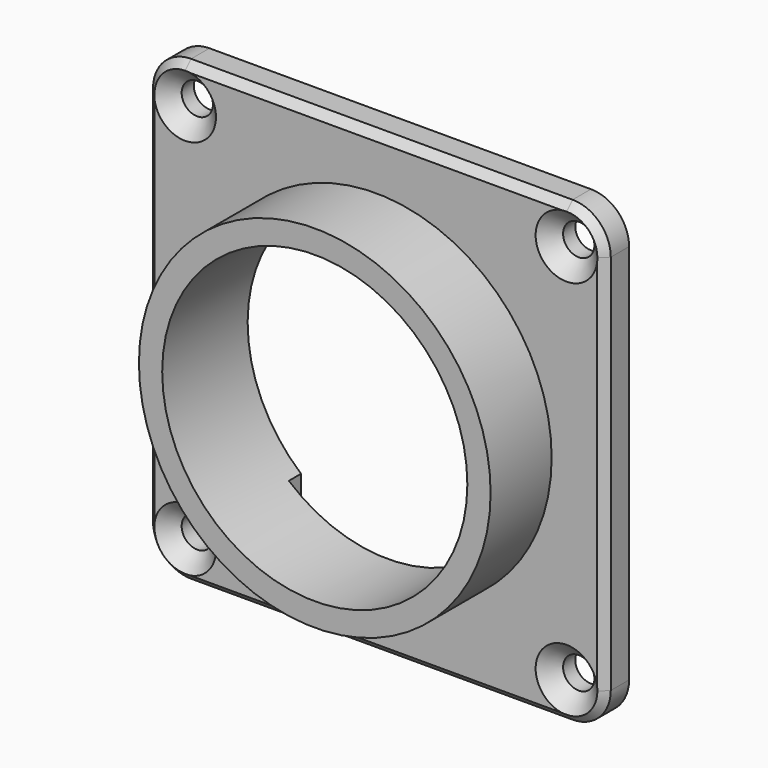
from build123d import *

# Parameters (mm, degrees)
F0_R          = 2.05
F0_R_2        = 20
F1_DEPTH      = 4
F2_R          = 1.95
F3_DEPTH      = 4
F4_SIZE       = 1
F5_R          = 23.05
F5_R_2        = 20
F6_DEPTH      = 10
F8_DEPTH      = 2
F9_R          = 0.8
F10_DEPTH     = 6
F11_SIZE      = 2
F12_T1_DEPTH  = 50
F12_T3_DEPTH  = 50
F12_T6_ANGLE  = 90
F12_T8_ANGLE  = 90
F12_T10_ANGLE = 90
F12_T12_ANGLE = 90


# Not quite as in the source:
# - a fillet or chamfer that OpenCascade refuses, or shapes differently, is made with other operations: its cross-section is extruded or revolved along the edge and cut away or added


with BuildPart() as f1:
    # F0 (on Front) → F1 (new body)
    with BuildSketch(Plane.XZ):
        with BuildLine():
            ThreePointArc((30, 25), (28.5355339059, 28.5355339059), (25, 30))
            Line((25, 30), (-25, 30))
            ThreePointArc((-25, 30), (-28.5355339059, 28.5355339059), (-30, 25))
            Line((-30, 25), (-30, -25))
            ThreePointArc((-30, -25), (-28.5355339059, -28.5355339059), (-25, -30))
            Line((-25, -30), (25, -30))
            ThreePointArc((25, -30), (28.5355339059, -28.5355339059), (30, -25))
            Line((30, -25), (30, 25))
        make_face()
        with Locations((-25, -25)):
            Circle(F0_R, mode=Mode.SUBTRACT)
        with Locations((25, -25)):
            Circle(F0_R, mode=Mode.SUBTRACT)
        Circle(F0_R_2, mode=Mode.SUBTRACT)
        with Locations((-25, 25)):
            Circle(F0_R, mode=Mode.SUBTRACT)
        with Locations((25, 25)):
            Circle(F0_R, mode=Mode.SUBTRACT)
    extrude(amount=F1_DEPTH)

    # F2 (on face) → F3 (join)
    with BuildSketch(Plane(origin=(0, 0, 0), x_dir=(-1, 0, 0), z_dir=(0, 1, 0))):
        with Locations((-19, 25)):
            Circle(F2_R)
        with Locations((19, 25)):
            Circle(F2_R)
        with Locations((19, -25)):
            Circle(F2_R)
        with Locations((-16, -25)):
            Circle(F2_R)
    extrude(amount=F3_DEPTH)

    # F4
    f4_edges = [f1.edges().sort_by_distance(p)[0] for p in [
        (17.95, 4, -25),
        (-17.05, 4, -25),
        (-17.05, 4, 25),
        (20.95, 4, 25),
    ]]
    chamfer(f4_edges, length=F4_SIZE)

    # F5 (on face) → F6 (join)
    with BuildSketch(Plane.XZ.offset(4)):
        Circle(F5_R)
        Circle(F5_R_2, mode=Mode.SUBTRACT)
    extrude(amount=F6_DEPTH)

    # F7 (on face) → F8 (cut)
    with BuildSketch(Plane(origin=(0, 0, 0), x_dir=(-1, 0, 0), z_dir=(0, 1, 0))):
        with BuildLine():
            ThreePointArc((13, -15.1986841536), (0, -20), (-13, -15.1986841536))
            Line((-13, -15.1986841536), (-13, -23))
            ThreePointArc((-13, -23), (-12.4142135624, -24.4142135624), (-11, -25))
            Line((-11, -25), (11, -25))
            ThreePointArc((11, -25), (12.4142135624, -24.4142135624), (13, -23))
            Line((13, -23), (13, -15.1986841536))
        make_face()
    extrude(amount=-F8_DEPTH, mode=Mode.SUBTRACT)

    # F9 (on face) → F10 (cut)
    with BuildSketch(Plane(origin=(0, -2, 0), x_dir=(-1, 0, 0), z_dir=(0, 1, 0))):
        with Locations((-11.4065121626, -18.2542352698)):
            Circle(F9_R)
        with Locations((11.4065121626, -18.2542352698)):
            Circle(F9_R)
    extrude(amount=-F10_DEPTH, mode=Mode.SUBTRACT)

    # F11
    f11_edges = [f1.edges().sort_by_distance(p)[0] for p in [
        (22.95, -4, 25),
        (-27.05, -4, 25),
        (-27.05, -4, -25),
        (22.95, -4, -25),
    ]]
    chamfer(f11_edges, length=F11_SIZE)

    # F12: chamfer of 1 on 8 edges, made by hand

    # F12_s2 → F12_t1 (cut)
    with BuildSketch(Plane.XY.offset(-25)):
        with BuildLine():
            Line((28.9717157288, -4.0282842712), (30.0282842712, -2.9717157288))
            Line((30.0282842712, -2.9717157288), (30.0482842712, -2.9717157288))
            ThreePointArc((30.0482842712, -2.9717157288), (30.02, -3.4858578644), (30.02, -4))
            Line((30.02, -4), (30, -4.02))
            ThreePointArc((30, -4.02), (29.4858578644, -4.02), (28.9717157288, -4.0482842712))
            Line((28.9717157288, -4.0482842712), (28.9717157288, -4.0282842712))
        make_face()
        with BuildLine():
            Line((-28.9717157288, -4.0282842712), (-30.0282842712, -2.9717157288))
            Line((-30.0282842712, -2.9717157288), (-30.0482842712, -2.9717157288))
            ThreePointArc((-30.0482842712, -2.9717157288), (-30.02, -3.4858578644), (-30.02, -4))
            Line((-30.02, -4), (-30, -4.02))
            ThreePointArc((-30, -4.02), (-29.4858578644, -4.02), (-28.9717157288, -4.0482842712))
            Line((-28.9717157288, -4.0482842712), (-28.9717157288, -4.0282842712))
        make_face()
    extrude(amount=F12_T1_DEPTH, mode=Mode.SUBTRACT)

    # F12_s4 → F12_t3 (cut)
    with BuildSketch(Plane.YZ.offset(-25)):
        with BuildLine():
            Line((-4.0282842712, 28.9717157288), (-2.9717157288, 30.0282842712))
            Line((-2.9717157288, 30.0282842712), (-2.9717157288, 30.0482842712))
            ThreePointArc((-2.9717157288, 30.0482842712), (-3.4858578644, 30.02), (-4, 30.02))
            Line((-4, 30.02), (-4.02, 30))
            ThreePointArc((-4.02, 30), (-4.02, 29.4858578644), (-4.0482842712, 28.9717157288))
            Line((-4.0482842712, 28.9717157288), (-4.0282842712, 28.9717157288))
        make_face()
        with BuildLine():
            Line((-4.0282842712, -28.9717157288), (-2.9717157288, -30.0282842712))
            Line((-2.9717157288, -30.0282842712), (-2.9717157288, -30.0482842712))
            ThreePointArc((-2.9717157288, -30.0482842712), (-3.4858578644, -30.02), (-4, -30.02))
            Line((-4, -30.02), (-4.02, -30))
            ThreePointArc((-4.02, -30), (-4.02, -29.4858578644), (-4.0482842712, -28.9717157288))
            Line((-4.0482842712, -28.9717157288), (-4.0282842712, -28.9717157288))
        make_face()
    extrude(amount=F12_T3_DEPTH, mode=Mode.SUBTRACT)

    # F12_s5 → F12_t6 (revolve, cut)
    with BuildSketch(Plane.XY.offset(25)):
        with BuildLine():
            Line((28.9717157288, -4.0282842712), (30.0282842712, -2.9717157288))
            Line((30.0282842712, -2.9717157288), (30.0482842712, -2.9717157288))
            ThreePointArc((30.0482842712, -2.9717157288), (30.02, -3.4858578644), (30.02, -4))
            Line((30.02, -4), (30, -4.02))
            ThreePointArc((30, -4.02), (29.4858578644, -4.02), (28.9717157288, -4.0482842712))
            Line((28.9717157288, -4.0482842712), (28.9717157288, -4.0282842712))
        make_face()
    revolve(axis=Axis((25, -4, 25), (0, -1, 0)), revolution_arc=F12_T6_ANGLE, mode=Mode.SUBTRACT)

    # F12_s7 → F12_t8 (revolve, cut)
    with BuildSketch(Plane.YZ.offset(-25)):
        with BuildLine():
            Line((-4.0282842712, 28.9717157288), (-2.9717157288, 30.0282842712))
            Line((-2.9717157288, 30.0282842712), (-2.9717157288, 30.0482842712))
            ThreePointArc((-2.9717157288, 30.0482842712), (-3.4858578644, 30.02), (-4, 30.02))
            Line((-4, 30.02), (-4.02, 30))
            ThreePointArc((-4.02, 30), (-4.02, 29.4858578644), (-4.0482842712, 28.9717157288))
            Line((-4.0482842712, 28.9717157288), (-4.0282842712, 28.9717157288))
        make_face()
    revolve(axis=Axis((-25, -4, 25), (0, -1, 0)), revolution_arc=F12_T8_ANGLE, mode=Mode.SUBTRACT)

    # F12_s9 → F12_t10 (revolve, cut)
    with BuildSketch(Plane.XY.offset(-25)):
        with BuildLine():
            Line((-28.9717157288, -4.0282842712), (-30.0282842712, -2.9717157288))
            Line((-30.0282842712, -2.9717157288), (-30.0482842712, -2.9717157288))
            ThreePointArc((-30.0482842712, -2.9717157288), (-30.02, -3.4858578644), (-30.02, -4))
            Line((-30.02, -4), (-30, -4.02))
            ThreePointArc((-30, -4.02), (-29.4858578644, -4.02), (-28.9717157288, -4.0482842712))
            Line((-28.9717157288, -4.0482842712), (-28.9717157288, -4.0282842712))
        make_face()
    revolve(axis=Axis((-25, -4, -25), (0, -1, 0)), revolution_arc=F12_T10_ANGLE, mode=Mode.SUBTRACT)

    # F12_s11 → F12_t12 (revolve, cut)
    with BuildSketch(Plane.YZ.offset(25)):
        with BuildLine():
            Line((-4.0282842712, -28.9717157288), (-2.9717157288, -30.0282842712))
            Line((-2.9717157288, -30.0282842712), (-2.9717157288, -30.0482842712))
            ThreePointArc((-2.9717157288, -30.0482842712), (-3.4858578644, -30.02), (-4, -30.02))
            Line((-4, -30.02), (-4.02, -30))
            ThreePointArc((-4.02, -30), (-4.02, -29.4858578644), (-4.0482842712, -28.9717157288))
            Line((-4.0482842712, -28.9717157288), (-4.0282842712, -28.9717157288))
        make_face()
    revolve(axis=Axis((25, -4, -25), (0, -1, 0)), revolution_arc=F12_T12_ANGLE, mode=Mode.SUBTRACT)


solid = f1.part
